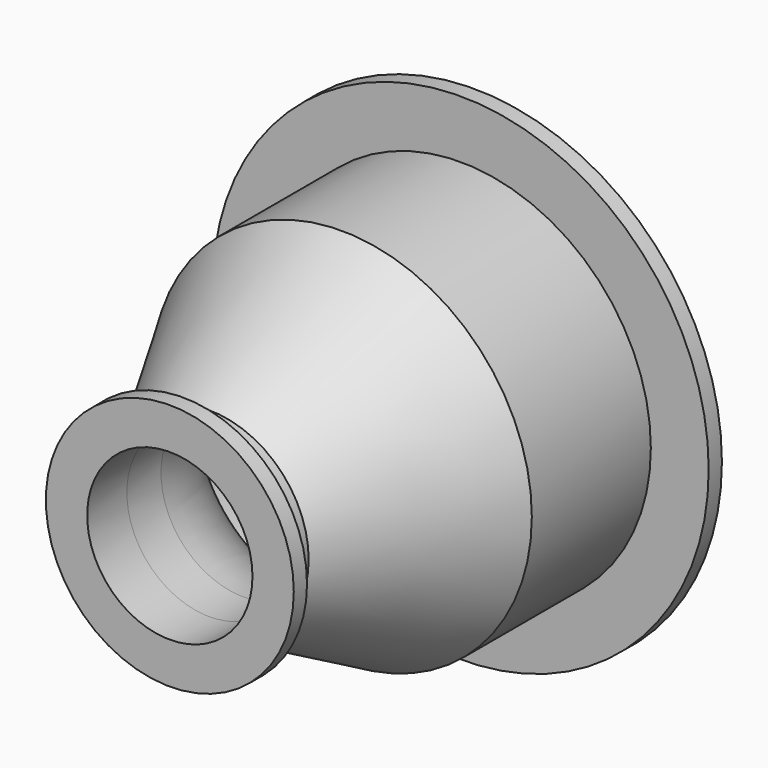
from build123d import *

# Parameters (mm, degrees)
F0_R      = 29.21
F0_R_2    = 25.4
F1_DEPTH  = 25.4
F0_R_3    = 38.1
F2_DEPTH  = 2.54
F5_R      = 29.21
F4_R      = 15.24
F7_R      = 15.24
F7_R_2    = 12.7
F8_DEPTH  = 7.62
F9_R      = 19.05
F9_R_2    = 15.24
F10_DEPTH = 2.54
F11_DEPTH = 57.658


# Not quite as in the source:
# - a fillet or chamfer that OpenCascade refuses, or shapes differently, is made with other operations: its cross-section is extruded or revolved along the edge and cut away or added


with BuildPart() as f1:
    # F0 (on Front) → F1 (new body)
    with BuildSketch(Plane.XZ):
        Circle(F0_R)
        Circle(F0_R_2, mode=Mode.SUBTRACT)
    extrude(amount=F1_DEPTH)

    # F0 (on Front) → F2 (join)
    with BuildSketch(Plane.XZ):
        Circle(F0_R_3)
        Circle(F0_R, mode=Mode.SUBTRACT)
    extrude(amount=F2_DEPTH)

    # F5 (on face) → F6 section 0
    with BuildSketch(Plane.XZ.offset(25.4)):
        Circle(F5_R)
    # F4 (on offset) → F6 section 1
    with BuildSketch(Plane.XZ.offset(50.8)):
        Circle(F4_R)
    loft()

    # F7 (on face) → F8 (join)
    with BuildSketch(Plane.XZ.offset(50.8)):
        Circle(F7_R)
        Circle(F7_R_2, mode=Mode.SUBTRACT)
    extrude(amount=F8_DEPTH)

    # F9 (on face) → F10 (join)
    with BuildSketch(Plane.XZ.offset(58.42)):
        Circle(F9_R)
        Circle(F9_R_2, mode=Mode.SUBTRACT)
    extrude(amount=-F10_DEPTH)

    # F11 (cut): a face of the model
    f11_faces = [f1.faces().sort_by_distance(p)[0] for p in [
        (0, -50.8, 0),
    ]]
    extrude(f11_faces, amount=-F11_DEPTH, mode=Mode.SUBTRACT)

    # F12: fillet of radius 20.32 on 1 edges, made by hand

    # F12_s1 → F12_t2 (revolve, cut)
    with BuildSketch(Plane.XY):
        with BuildLine():
            ThreePointArc((25.4, -25.4), (16.171546065, -32.8779188315), (12.7, -44.2371441572))
            Line((12.7, -44.2371441572), (12.7, -25.4))
            Line((12.7, -25.4), (25.4, -25.4))
        make_face()
    revolve(axis=Axis((0, -25.4, 0), (0, -1, 0)), mode=Mode.SUBTRACT)


solid = f1.part
